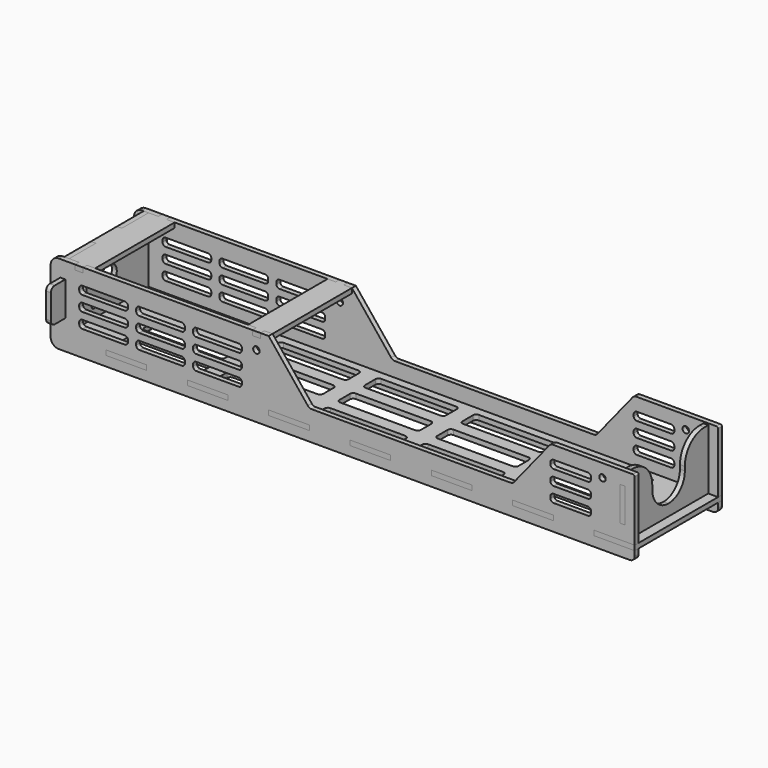
from build123d import *

# Parameters (mm, degrees)
F1_W      = 25
F1_H      = 3
F2_DEPTH  = 3
F3_W      = 25
F3_H      = 3
F3_W_2    = 3
F3_H_2    = 21
F3_R      = 2
F4_DEPTH  = 3
F6_R      = 1.65
F6_R_2    = 6.1
F7_DEPTH  = 3
F10_DEPTH = 3
F8_W      = 3
F8_H      = 21
F11_DEPTH = 3


# Not quite as in the source:
# - a feature names something its author has since deleted; it is built from what else it names


with BuildPart() as f2:
    # F1 (on Top) → F2 (new body)
    with BuildSketch(Plane.XY):
        Polygon((0, 10), (0, 0), (0, -10), (0, -30.5), (25, -30.5), (50, -30.5), (75, -30.5), (100, -30.5), (125, -30.5), (150, -30.5), (175, -30.5), (200, -30.5), (225, -30.5), (250, -30.5), (275, -30.5), (300, -30.5), (325, -30.5), (350, -30.5), (350, 0), (350, 30.5), (325, 30.5), (300, 30.5), (275, 30.5), (250, 30.5), (225, 30.5), (200, 30.5), (175, 30.5), (150, 30.5), (125, 30.5), (100, 30.5), (75, 30.5), (50, 30.5), (25, 30.5), (0, 30.5), align=None)
        with BuildLine():
            ThreePointArc((73, -13.5), (74.4142135624, -14.0857864376), (75, -15.5))
            Line((75, -15.5), (75, -23.5))
            ThreePointArc((75, -23.5), (74.4142135624, -24.9142135624), (73, -25.5))
            Line((73, -25.5), (27, -25.5))
            ThreePointArc((27, -25.5), (25.5857864376, -24.9142135624), (25, -23.5))
            Line((25, -23.5), (25, -15.5))
            ThreePointArc((25, -15.5), (25.5857864376, -14.0857864376), (27, -13.5))
            Line((27, -13.5), (73, -13.5))
        make_face(mode=Mode.SUBTRACT)
        with BuildLine():
            ThreePointArc((87, -25.5), (85.5857864376, -24.9142135624), (85, -23.5))
            Line((85, -23.5), (85, -15.5))
            ThreePointArc((85, -15.5), (85.5857864376, -14.0857864376), (87, -13.5))
            Line((87, -13.5), (133, -13.5))
            ThreePointArc((133, -13.5), (134.4142135624, -14.0857864376), (135, -15.5))
            Line((135, -15.5), (135, -23.5))
            ThreePointArc((135, -23.5), (134.4142135624, -24.9142135624), (133, -25.5))
            Line((133, -25.5), (87, -25.5))
        make_face(mode=Mode.SUBTRACT)
        with BuildLine():
            ThreePointArc((193, -13.5), (194.4142135624, -14.0857864376), (195, -15.5))
            Line((195, -15.5), (195, -23.5))
            ThreePointArc((195, -23.5), (194.4142135624, -24.9142135624), (193, -25.5))
            Line((193, -25.5), (147, -25.5))
            ThreePointArc((147, -25.5), (145.5857864376, -24.9142135624), (145, -23.5))
            Line((145, -23.5), (145, -15.5))
            ThreePointArc((145, -15.5), (145.5857864376, -14.0857864376), (147, -13.5))
            Line((147, -13.5), (193, -13.5))
        make_face(mode=Mode.SUBTRACT)
        with BuildLine():
            ThreePointArc((207, -25.5), (205.5857864376, -24.9142135624), (205, -23.5))
            Line((205, -23.5), (205, -15.5))
            ThreePointArc((205, -15.5), (205.5857864376, -14.0857864376), (207, -13.5))
            Line((207, -13.5), (253, -13.5))
            ThreePointArc((253, -13.5), (254.4142135624, -14.0857864376), (255, -15.5))
            Line((255, -15.5), (255, -23.5))
            ThreePointArc((255, -23.5), (254.4142135624, -24.9142135624), (253, -25.5))
            Line((253, -25.5), (207, -25.5))
        make_face(mode=Mode.SUBTRACT)
        with BuildLine():
            ThreePointArc((267, -25.5), (265.5857864376, -24.9142135624), (265, -23.5))
            Line((265, -23.5), (265, -15.5))
            ThreePointArc((265, -15.5), (265.5857864376, -14.0857864376), (267, -13.5))
            Line((267, -13.5), (313, -13.5))
            ThreePointArc((313, -13.5), (314.4142135624, -14.0857864376), (315, -15.5))
            Line((315, -15.5), (315, -23.5))
            ThreePointArc((315, -23.5), (314.4142135624, -24.9142135624), (313, -25.5))
            Line((313, -25.5), (267, -25.5))
        make_face(mode=Mode.SUBTRACT)
        with BuildLine():
            Line((25, -4), (25, 0))
            Line((25, 0), (25, 4))
            ThreePointArc((25, 4), (25.5857864376, 5.4142135624), (27, 6))
            Line((27, 6), (73, 6))
            ThreePointArc((73, 6), (74.4142135624, 5.4142135624), (75, 4))
            Line((75, 4), (75, 0))
            Line((75, 0), (75, -4))
            ThreePointArc((75, -4), (74.4142135624, -5.4142135624), (73, -6))
            Line((73, -6), (27, -6))
            ThreePointArc((27, -6), (25.5857864376, -5.4142135624), (25, -4))
        make_face(mode=Mode.SUBTRACT)
        with BuildLine():
            ThreePointArc((85, 4), (85.5857864376, 5.4142135624), (87, 6))
            Line((87, 6), (133, 6))
            ThreePointArc((133, 6), (134.4142135624, 5.4142135624), (135, 4))
            Line((135, 4), (135, 0))
            Line((135, 0), (135, -4))
            ThreePointArc((135, -4), (134.4142135624, -5.4142135624), (133, -6))
            Line((133, -6), (87, -6))
            ThreePointArc((87, -6), (85.5857864376, -5.4142135624), (85, -4))
            Line((85, -4), (85, 0))
            Line((85, 0), (85, 4))
        make_face(mode=Mode.SUBTRACT)
        with BuildLine():
            ThreePointArc((145, 4), (145.5857864376, 5.4142135624), (147, 6))
            Line((147, 6), (193, 6))
            ThreePointArc((193, 6), (194.4142135624, 5.4142135624), (195, 4))
            Line((195, 4), (195, 0))
            Line((195, 0), (195, -4))
            ThreePointArc((195, -4), (194.4142135624, -5.4142135624), (193, -6))
            Line((193, -6), (147, -6))
            ThreePointArc((147, -6), (145.5857864376, -5.4142135624), (145, -4))
            Line((145, -4), (145, 0))
            Line((145, 0), (145, 4))
        make_face(mode=Mode.SUBTRACT)
        with BuildLine():
            ThreePointArc((25, 23.5), (25.5857864376, 24.9142135624), (27, 25.5))
            Line((27, 25.5), (73, 25.5))
            ThreePointArc((73, 25.5), (74.4142135624, 24.9142135624), (75, 23.5))
            Line((75, 23.5), (75, 15.5))
            ThreePointArc((75, 15.5), (74.4142135624, 14.0857864376), (73, 13.5))
            Line((73, 13.5), (27, 13.5))
            ThreePointArc((27, 13.5), (25.5857864376, 14.0857864376), (25, 15.5))
            Line((25, 15.5), (25, 23.5))
        make_face(mode=Mode.SUBTRACT)
        with BuildLine():
            Line((135, 23.5), (135, 15.5))
            ThreePointArc((135, 15.5), (134.4142135624, 14.0857864376), (133, 13.5))
            Line((133, 13.5), (87, 13.5))
            ThreePointArc((87, 13.5), (85.5857864376, 14.0857864376), (85, 15.5))
            Line((85, 15.5), (85, 23.5))
            ThreePointArc((85, 23.5), (85.5857864376, 24.9142135624), (87, 25.5))
            Line((87, 25.5), (133, 25.5))
            ThreePointArc((133, 25.5), (134.4142135624, 24.9142135624), (135, 23.5))
        make_face(mode=Mode.SUBTRACT)
        with BuildLine():
            Line((195, 23.5), (195, 15.5))
            ThreePointArc((195, 15.5), (194.4142135624, 14.0857864376), (193, 13.5))
            Line((193, 13.5), (147, 13.5))
            ThreePointArc((147, 13.5), (145.5857864376, 14.0857864376), (145, 15.5))
            Line((145, 15.5), (145, 23.5))
            ThreePointArc((145, 23.5), (145.5857864376, 24.9142135624), (147, 25.5))
            Line((147, 25.5), (193, 25.5))
            ThreePointArc((193, 25.5), (194.4142135624, 24.9142135624), (195, 23.5))
        make_face(mode=Mode.SUBTRACT)
        with BuildLine():
            ThreePointArc((205, 4), (205.5857864376, 5.4142135624), (207, 6))
            Line((207, 6), (253, 6))
            ThreePointArc((253, 6), (254.4142135624, 5.4142135624), (255, 4))
            Line((255, 4), (255, 0))
            Line((255, 0), (255, -4))
            ThreePointArc((255, -4), (254.4142135624, -5.4142135624), (253, -6))
            Line((253, -6), (207, -6))
            ThreePointArc((207, -6), (205.5857864376, -5.4142135624), (205, -4))
            Line((205, -4), (205, 0))
            Line((205, 0), (205, 4))
        make_face(mode=Mode.SUBTRACT)
        with BuildLine():
            ThreePointArc((265, 4), (265.5857864376, 5.4142135624), (267, 6))
            Line((267, 6), (313, 6))
            ThreePointArc((313, 6), (314.4142135624, 5.4142135624), (315, 4))
            Line((315, 4), (315, 0))
            Line((315, 0), (315, -4))
            ThreePointArc((315, -4), (314.4142135624, -5.4142135624), (313, -6))
            Line((313, -6), (267, -6))
            ThreePointArc((267, -6), (265.5857864376, -5.4142135624), (265, -4))
            Line((265, -4), (265, 0))
            Line((265, 0), (265, 4))
        make_face(mode=Mode.SUBTRACT)
        Polygon((344, 10), (344, 0), (344, -10), (341, -10), (341, 10), align=None, mode=Mode.SUBTRACT)
        with BuildLine():
            Line((255, 23.5), (255, 15.5))
            ThreePointArc((255, 15.5), (254.4142135624, 14.0857864376), (253, 13.5))
            Line((253, 13.5), (207, 13.5))
            ThreePointArc((207, 13.5), (205.5857864376, 14.0857864376), (205, 15.5))
            Line((205, 15.5), (205, 23.5))
            ThreePointArc((205, 23.5), (205.5857864376, 24.9142135624), (207, 25.5))
            Line((207, 25.5), (253, 25.5))
            ThreePointArc((253, 25.5), (254.4142135624, 24.9142135624), (255, 23.5))
        make_face(mode=Mode.SUBTRACT)
        with BuildLine():
            Line((315, 23.5), (315, 15.5))
            ThreePointArc((315, 15.5), (314.4142135624, 14.0857864376), (313, 13.5))
            Line((313, 13.5), (267, 13.5))
            ThreePointArc((267, 13.5), (265.5857864376, 14.0857864376), (265, 15.5))
            Line((265, 15.5), (265, 23.5))
            ThreePointArc((265, 23.5), (265.5857864376, 24.9142135624), (267, 25.5))
            Line((267, 25.5), (313, 25.5))
            ThreePointArc((313, 25.5), (314.4142135624, 24.9142135624), (315, 23.5))
        make_face(mode=Mode.SUBTRACT)
        with Locations((37.5, 32)):
            Rectangle(F1_W, F1_H)
        with Locations((87.5, 32)):
            Rectangle(F1_W, F1_H)
        with Locations((137.5, 32)):
            Rectangle(F1_W, F1_H)
        with Locations((187.5, 32)):
            Rectangle(F1_W, F1_H)
        with Locations((237.5, 32)):
            Rectangle(F1_W, F1_H)
        with Locations((37.5, -32)):
            Rectangle(F1_W, F1_H)
        with Locations((87.5, -32)):
            Rectangle(F1_W, F1_H)
        with Locations((137.5, -32)):
            Rectangle(F1_W, F1_H)
        with Locations((187.5, -32)):
            Rectangle(F1_W, F1_H)
        with Locations((237.5, -32)):
            Rectangle(F1_W, F1_H)
        with Locations((287.5, 32)):
            Rectangle(F1_W, F1_H)
        with Locations((337.5, 32)):
            Rectangle(F1_W, F1_H)
        with Locations((287.5, -32)):
            Rectangle(F1_W, F1_H)
        with Locations((337.5, -32)):
            Rectangle(F1_W, F1_H)
        Polygon((0, -10), (0, 0), (0, 10), (-3, 10), (-3, 0), (-3, -10), align=None)
    extrude(amount=F2_DEPTH)


with BuildPart() as f4:
    # F3 (on face) → F4 (new body)
    with BuildSketch(Plane.XZ.offset(33.5)):
        with BuildLine():
            Line((350, 0), (325, 0))
            Line((325, 0), (325, 3))
            Line((325, 3), (350, 3))
            Line((350, 3), (350, 40))
            ThreePointArc((350, 40), (349.7071067812, 40.7071067812), (349, 41))
            Line((349, 41), (299.8217369842, 41))
            ThreePointArc((299.8217369842, 41), (298.5274750441, 40.7064526655), (297.4864978658, 39.8832573536))
            Line((297.4864978658, 39.8832573536), (275.9005989084, 13.1167426464))
            ThreePointArc((275.9005989084, 13.1167426464), (274.8596217301, 12.2935473345), (273.56535979, 12))
            Line((273.56535979, 12), (151.43464021, 12))
            ThreePointArc((151.43464021, 12), (150.1403782699, 12.2935473345), (149.0994010916, 13.1167426464))
            Line((149.0994010916, 13.1167426464), (125, 43))
            Line((125, 43), (120, 43))
            Line((120, 43), (120, 40))
            Line((120, 40), (115, 40))
            Line((115, 40), (115, 43))
            Line((115, 43), (11, 43))
            Line((11, 43), (11, 40))
            Line((11, 40), (6, 40))
            Line((6, 40), (6, 43))
            Line((6, 43), (0, 43))
            Line((0, 43), (-4, 43))
            ThreePointArc((-4, 43), (-7.5355339059, 41.5355339059), (-9, 38))
            Line((-9, 38), (-9, -1))
            ThreePointArc((-9, -1), (-7.5355339059, -4.5355339059), (-4, -6))
            Line((-4, -6), (0, -6))
            Line((0, -6), (347, -6))
            ThreePointArc((347, -6), (349.1213203436, -5.1213203436), (350, -3))
            Line((350, -3), (350, 0))
        make_face()
        with Locations((37.5, 1.5)):
            Rectangle(F3_W, F3_H, mode=Mode.SUBTRACT)
        with Locations((87.5, 1.5)):
            Rectangle(F3_W, F3_H, mode=Mode.SUBTRACT)
        with Locations((137.5, 1.5)):
            Rectangle(F3_W, F3_H, mode=Mode.SUBTRACT)
        with BuildLine():
            ThreePointArc((8.5543720052, 12.6), (9.1401584428, 14.0142135624), (10.5543720052, 14.6))
            Line((10.5543720052, 14.6), (36.5543720052, 14.6))
            ThreePointArc((36.5543720052, 14.6), (37.9685855675, 14.0142135624), (38.5543720052, 12.6))
            Line((38.5543720052, 12.6), (38.5543720052, 11.6))
            ThreePointArc((38.5543720052, 11.6), (37.9685855675, 10.1857864376), (36.5543720052, 9.6))
            Line((36.5543720052, 9.6), (10.5543720052, 9.6))
            ThreePointArc((10.5543720052, 9.6), (9.1401584428, 10.1857864376), (8.5543720052, 11.6))
            Line((8.5543720052, 11.6), (8.5543720052, 12.6))
        make_face(mode=Mode.SUBTRACT)
        with BuildLine():
            ThreePointArc((43.5543720052, 12.6), (44.1401584428, 14.0142135624), (45.5543720052, 14.6))
            Line((45.5543720052, 14.6), (71.5543720052, 14.6))
            ThreePointArc((71.5543720052, 14.6), (72.9685855675, 14.0142135624), (73.5543720052, 12.6))
            Line((73.5543720052, 12.6), (73.5543720052, 11.6))
            ThreePointArc((73.5543720052, 11.6), (72.9685855675, 10.1857864376), (71.5543720052, 9.6))
            Line((71.5543720052, 9.6), (45.5543720052, 9.6))
            ThreePointArc((45.5543720052, 9.6), (44.1401584428, 10.1857864376), (43.5543720052, 11.6))
            Line((43.5543720052, 11.6), (43.5543720052, 12.6))
        make_face(mode=Mode.SUBTRACT)
        with BuildLine():
            ThreePointArc((78.5543720052, 12.6), (79.1401584428, 14.0142135624), (80.5543720052, 14.6))
            Line((80.5543720052, 14.6), (106.5543720052, 14.6))
            ThreePointArc((106.5543720052, 14.6), (107.9685855675, 14.0142135624), (108.5543720052, 12.6))
            Line((108.5543720052, 12.6), (108.5543720052, 11.6))
            ThreePointArc((108.5543720052, 11.6), (107.9685855675, 10.1857864376), (106.5543720052, 9.6))
            Line((106.5543720052, 9.6), (80.5543720052, 9.6))
            ThreePointArc((80.5543720052, 9.6), (79.1401584428, 10.1857864376), (78.5543720052, 11.6))
            Line((78.5543720052, 11.6), (78.5543720052, 12.6))
        make_face(mode=Mode.SUBTRACT)
        with Locations((187.5, 1.5)):
            Rectangle(F3_W, F3_H, mode=Mode.SUBTRACT)
        with Locations((237.5, 1.5)):
            Rectangle(F3_W, F3_H, mode=Mode.SUBTRACT)
        with Locations((287.5, 1.5)):
            Rectangle(F3_W, F3_H, mode=Mode.SUBTRACT)
        with BuildLine():
            ThreePointArc((323.1663644314, 11.6), (322.5805779938, 10.1857864376), (321.1663644314, 9.6))
            Line((321.1663644314, 9.6), (300.1663644314, 9.6))
            ThreePointArc((300.1663644314, 9.6), (298.752150869, 10.1857864376), (298.1663644314, 11.6))
            Line((298.1663644314, 11.6), (298.1663644314, 12.6))
            ThreePointArc((298.1663644314, 12.6), (298.752150869, 14.0142135624), (300.1663644314, 14.6))
            Line((300.1663644314, 14.6), (321.1663644314, 14.6))
            ThreePointArc((321.1663644314, 14.6), (322.5805779938, 14.0142135624), (323.1663644314, 12.6))
            Line((323.1663644314, 12.6), (323.1663644314, 11.6))
        make_face(mode=Mode.SUBTRACT)
        with BuildLine():
            ThreePointArc((8.5543720052, 21.8), (9.1401584428, 23.2142135624), (10.5543720052, 23.8))
            Line((10.5543720052, 23.8), (36.5543720052, 23.8))
            ThreePointArc((36.5543720052, 23.8), (37.9685855675, 23.2142135624), (38.5543720052, 21.8))
            Line((38.5543720052, 21.8), (38.5543720052, 20.8))
            ThreePointArc((38.5543720052, 20.8), (37.9685855675, 19.3857864376), (36.5543720052, 18.8))
            Line((36.5543720052, 18.8), (10.5543720052, 18.8))
            ThreePointArc((10.5543720052, 18.8), (9.1401584428, 19.3857864376), (8.5543720052, 20.8))
            Line((8.5543720052, 20.8), (8.5543720052, 21.8))
        make_face(mode=Mode.SUBTRACT)
        with Locations((-1.5, 22.5)):
            Rectangle(F3_W_2, F3_H_2, mode=Mode.SUBTRACT)
        with BuildLine():
            ThreePointArc((43.5543720052, 21.8), (44.1401584428, 23.2142135624), (45.5543720052, 23.8))
            Line((45.5543720052, 23.8), (71.5543720052, 23.8))
            ThreePointArc((71.5543720052, 23.8), (72.9685855675, 23.2142135624), (73.5543720052, 21.8))
            Line((73.5543720052, 21.8), (73.5543720052, 20.8))
            ThreePointArc((73.5543720052, 20.8), (72.9685855675, 19.3857864376), (71.5543720052, 18.8))
            Line((71.5543720052, 18.8), (45.5543720052, 18.8))
            ThreePointArc((45.5543720052, 18.8), (44.1401584428, 19.3857864376), (43.5543720052, 20.8))
            Line((43.5543720052, 20.8), (43.5543720052, 21.8))
        make_face(mode=Mode.SUBTRACT)
        with BuildLine():
            ThreePointArc((8.5543720052, 31), (9.1401584428, 32.4142135624), (10.5543720052, 33))
            Line((10.5543720052, 33), (36.5543720052, 33))
            ThreePointArc((36.5543720052, 33), (37.9685855675, 32.4142135624), (38.5543720052, 31))
            Line((38.5543720052, 31), (38.5543720052, 30))
            ThreePointArc((38.5543720052, 30), (37.9685855675, 28.5857864376), (36.5543720052, 28))
            Line((36.5543720052, 28), (10.5543720052, 28))
            ThreePointArc((10.5543720052, 28), (9.1401584428, 28.5857864376), (8.5543720052, 30))
            Line((8.5543720052, 30), (8.5543720052, 31))
        make_face(mode=Mode.SUBTRACT)
        with BuildLine():
            ThreePointArc((43.5543720052, 31), (44.1401584428, 32.4142135624), (45.5543720052, 33))
            Line((45.5543720052, 33), (71.5543720052, 33))
            ThreePointArc((71.5543720052, 33), (72.9685855675, 32.4142135624), (73.5543720052, 31))
            Line((73.5543720052, 31), (73.5543720052, 30))
            ThreePointArc((73.5543720052, 30), (72.9685855675, 28.5857864376), (71.5543720052, 28))
            Line((71.5543720052, 28), (45.5543720052, 28))
            ThreePointArc((45.5543720052, 28), (44.1401584428, 28.5857864376), (43.5543720052, 30))
            Line((43.5543720052, 30), (43.5543720052, 31))
        make_face(mode=Mode.SUBTRACT)
        with BuildLine():
            ThreePointArc((78.5543720052, 21.8), (79.1401584428, 23.2142135624), (80.5543720052, 23.8))
            Line((80.5543720052, 23.8), (106.5543720052, 23.8))
            ThreePointArc((106.5543720052, 23.8), (107.9685855675, 23.2142135624), (108.5543720052, 21.8))
            Line((108.5543720052, 21.8), (108.5543720052, 20.8))
            ThreePointArc((108.5543720052, 20.8), (107.9685855675, 19.3857864376), (106.5543720052, 18.8))
            Line((106.5543720052, 18.8), (80.5543720052, 18.8))
            ThreePointArc((80.5543720052, 18.8), (79.1401584428, 19.3857864376), (78.5543720052, 20.8))
            Line((78.5543720052, 20.8), (78.5543720052, 21.8))
        make_face(mode=Mode.SUBTRACT)
        with BuildLine():
            ThreePointArc((78.5543720052, 31), (79.1401584428, 32.4142135624), (80.5543720052, 33))
            Line((80.5543720052, 33), (106.5543720052, 33))
            ThreePointArc((106.5543720052, 33), (107.9685855675, 32.4142135624), (108.5543720052, 31))
            Line((108.5543720052, 31), (108.5543720052, 30))
            ThreePointArc((108.5543720052, 30), (107.9685855675, 28.5857864376), (106.5543720052, 28))
            Line((106.5543720052, 28), (80.5543720052, 28))
            ThreePointArc((80.5543720052, 28), (79.1401584428, 28.5857864376), (78.5543720052, 30))
            Line((78.5543720052, 30), (78.5543720052, 31))
        make_face(mode=Mode.SUBTRACT)
        with Locations((117.475, 33)):
            Circle(F3_R, mode=Mode.SUBTRACT)
        with BuildLine():
            ThreePointArc((323.1663644314, 20.8), (322.5805779938, 19.3857864376), (321.1663644314, 18.8))
            Line((321.1663644314, 18.8), (300.1663644314, 18.8))
            ThreePointArc((300.1663644314, 18.8), (298.752150869, 19.3857864376), (298.1663644314, 20.8))
            Line((298.1663644314, 20.8), (298.1663644314, 21.8))
            ThreePointArc((298.1663644314, 21.8), (298.752150869, 23.2142135624), (300.1663644314, 23.8))
            Line((300.1663644314, 23.8), (321.1663644314, 23.8))
            ThreePointArc((321.1663644314, 23.8), (322.5805779938, 23.2142135624), (323.1663644314, 21.8))
            Line((323.1663644314, 21.8), (323.1663644314, 20.8))
        make_face(mode=Mode.SUBTRACT)
        with Locations((342.5, 22.5)):
            Rectangle(F3_W_2, F3_H_2, mode=Mode.SUBTRACT)
        with BuildLine():
            Line((300.1663644314, 33), (321.1663644314, 33))
            ThreePointArc((321.1663644314, 33), (322.5805779938, 32.4142135624), (323.1663644314, 31))
            Line((323.1663644314, 31), (323.1663644314, 30))
            ThreePointArc((323.1663644314, 30), (322.5805779938, 28.5857864376), (321.1663644314, 28))
            Line((321.1663644314, 28), (300.1663644314, 28))
            ThreePointArc((300.1663644314, 28), (298.752150869, 28.5857864376), (298.1663644314, 30))
            Line((298.1663644314, 30), (298.1663644314, 31))
            ThreePointArc((298.1663644314, 31), (298.752150869, 32.4142135624), (300.1663644314, 33))
        make_face(mode=Mode.SUBTRACT)
        with Locations((330.2, 33)):
            Circle(F3_R, mode=Mode.SUBTRACT)
    extrude(amount=-F4_DEPTH)


with BuildPart() as f5_1:
    # F5: instance of F4
    add(f4.part.mirror(Plane.XZ))


with BuildPart() as f7:
    # F6 (on face) → F7 (new body)
    with BuildSketch(Plane(origin=(-3, 0, 0), x_dir=(0, -1, 0), z_dir=(-1, 0, 0))):
        with BuildLine():
            Line((10, 3), (10, 0))
            Line((10, 0), (30.5, 0))
            Line((30.5, 0), (30.5, 3))
            Line((30.5, 3), (30.5, 12))
            Line((30.5, 12), (33.5, 12))
            Line((33.5, 12), (41.5, 12))
            ThreePointArc((41.5, 12), (43.6213203436, 12.8786796564), (44.5, 15))
            Line((44.5, 15), (44.5, 30.2))
            ThreePointArc((44.5, 30.2), (43.6798989873, 32.1798989873), (41.7, 33))
            Line((41.7, 33), (33.5, 33))
            Line((33.5, 33), (30.5, 33))
            Line((30.5, 33), (30.5, 43))
            Line((30.5, 43), (10, 43))
            Line((10, 43), (10, 40))
            Line((10, 40), (-10, 40))
            Line((-10, 40), (-10, 43))
            Line((-10, 43), (-30.5, 43))
            Line((-30.5, 43), (-30.5, 33))
            Line((-30.5, 33), (-33.5, 33))
            Line((-33.5, 33), (-41.5, 33))
            ThreePointArc((-41.5, 33), (-43.6213203436, 32.1213203436), (-44.5, 30))
            Line((-44.5, 30), (-44.5, 15))
            ThreePointArc((-44.5, 15), (-43.6213203436, 12.8786796564), (-41.5, 12))
            Line((-41.5, 12), (-33.5, 12))
            Line((-33.5, 12), (-30.5, 12))
            Line((-30.5, 12), (-30.5, 3))
            Line((-30.5, 3), (-30.5, 0))
            Line((-30.5, 0), (-10, 0))
            Line((-10, 0), (-10, 3))
            Line((-10, 3), (10, 3))
        make_face()
        with Locations((-11.575, 9.925)):
            Circle(F6_R, mode=Mode.SUBTRACT)
        with Locations((11.575, 9.925)):
            Circle(F6_R, mode=Mode.SUBTRACT)
        with Locations((-11.575, 33.075)):
            Circle(F6_R, mode=Mode.SUBTRACT)
        with Locations((0.0125758201, 21.5)):
            Circle(F6_R_2, mode=Mode.SUBTRACT)
        with BuildLine():
            ThreePointArc((17.0263148248, 23.5864448845), (17.6121012624, 25.0006584469), (19.0263148248, 25.5864448845))
            Line((19.0263148248, 25.5864448845), (24.5, 25.5864448845))
            ThreePointArc((24.5, 25.5864448845), (25.9142135624, 25.0006584469), (26.5, 23.5864448845))
            Line((26.5, 23.5864448845), (26.5, 19.4135551155))
            ThreePointArc((26.5, 19.4135551155), (25.9142135624, 17.9993415531), (24.5, 17.4135551155))
            Line((24.5, 17.4135551155), (19.0263148248, 17.4135551155))
            ThreePointArc((19.0263148248, 17.4135551155), (17.6121012624, 17.9993415531), (17.0263148248, 19.4135551155))
            Line((17.0263148248, 19.4135551155), (17.0263148248, 23.5864448845))
        make_face(mode=Mode.SUBTRACT)
        with Locations((11.575, 33.075)):
            Circle(F6_R, mode=Mode.SUBTRACT)
    extrude(amount=-F7_DEPTH)


with BuildPart() as f10:
    # F9 (on face) → F10 (new body)
    with BuildSketch(Plane.XY.offset(43)):
        Polygon((11, 30.5), (11, 33.5), (6, 33.5), (6, 30.5), (0, 30.5), (0, 10), (-3, 10), (-3, -10), (0, -10), (0, -30.5), (6, -30.5), (6, -33.5), (11, -33.5), (11, -30.5), (16, -30.5), (16, 30.5), align=None)
    extrude(amount=-F10_DEPTH)


with BuildPart() as f10b:
    # F9 (on face) → F10, piece 2 (new body)
    with BuildSketch(Plane.XY.offset(43)):
        Polygon((120, 30.5), (120, 33.5), (115, 33.5), (115, 30.5), (110, 30.5), (110, -30.5), (115, -30.5), (115, -33.5), (120, -33.5), (120, -30.5), (125, -30.5), (125, 30.5), align=None)
    extrude(amount=-F10_DEPTH)


with BuildPart() as f11:
    # F8 (on face) → F11 (new body)
    with BuildSketch(Plane.YZ.offset(341)):
        with Locations((-32, 22.5)):
            Rectangle(F8_W, F8_H)
        with BuildLine():
            Line((30.5, 12), (33.5, 12))
            Line((33.5, 12), (33.5, 33))
            Line((33.5, 33), (30.5, 33))
            Line((30.5, 33), (30.5, 40))
            Line((30.5, 40), (27.5, 40))
            ThreePointArc((27.5, 40), (16.8933982822, 35.6066017178), (12.5, 25))
            Line((12.5, 25), (12.5, 22.5))
            ThreePointArc((12.5, 22.5), (8.8388347648, 13.6611652352), (0, 10))
            ThreePointArc((0, 10), (-8.8388347648, 13.6611652352), (-12.5, 22.5))
            Line((-12.5, 22.5), (-12.5, 25))
            ThreePointArc((-12.5, 25), (-16.8933982822, 35.6066017178), (-27.5, 40))
            Line((-27.5, 40), (-30.5, 40))
            Line((-30.5, 40), (-30.5, 33))
            Line((-30.5, 33), (-30.5, 12))
            Line((-30.5, 12), (-30.5, 3))
            Line((-30.5, 3), (-27.5, 3))
            Line((-27.5, 3), (-10, 3))
            Line((-10, 3), (-10, 0))
            Line((-10, 0), (0, 0))
            Line((0, 0), (10, 0))
            Line((10, 0), (10, 3))
            Line((10, 3), (27.5, 3))
            Line((27.5, 3), (30.5, 3))
            Line((30.5, 3), (30.5, 12))
        make_face()
    extrude(amount=F11_DEPTH)


solid = Compound([f2.part, f4.part, f5_1.part, f7.part, f10.part, f10b.part, f11.part])
